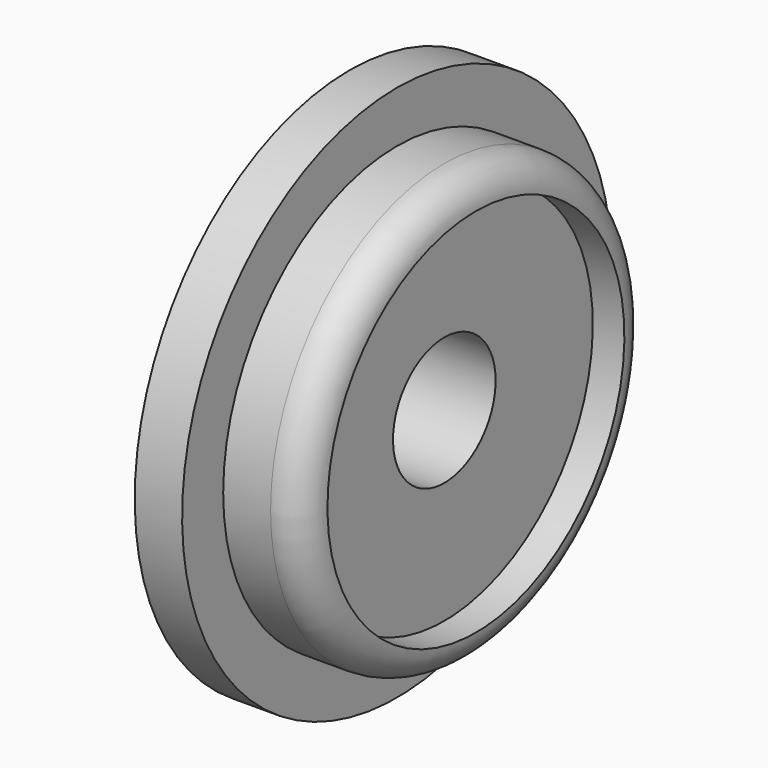
from build123d import *

# Parameters (mm, degrees)
F2_R = 1.99999


# Not quite as in the source:
# - a fillet or chamfer is up to 0.001 mm smaller than in the source, because OpenCascade refuses the exact size


with BuildPart() as f1:
    # F0 (on Front) → F1 (revolve)
    with BuildSketch(Plane.XZ):
        Polygon((0, 17), (0, 4.06), (6, 4.06), (6, 11.75), (8, 11.75), (8, 13.75), (3, 13.75), (3, 17), align=None)
    revolve(axis=Axis((3.2099459786, 0, 0), (1, 0, 0)))

    # F2 (radius 2 in the source; OpenCascade refuses exactly that, so slightly less here)
    f2_edges = [f1.edges().sort_by_distance(p)[0] for p in [
        (8, 0, -13.75),
    ]]
    fillet(f2_edges, radius=F2_R)


solid = f1.part
